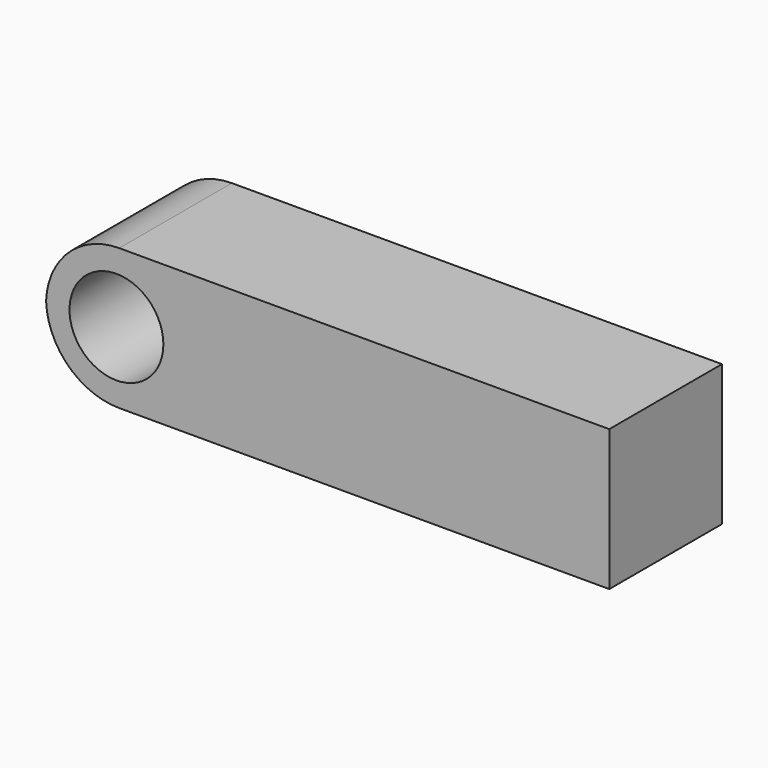
from build123d import *

# Parameters (mm, degrees)
F0_W        = 76.2
F0_H        = 19.05
F1_DEPTH    = 19.05
F3_D        = 12.7
F4_T1_DEPTH = 68.58


# Not quite as in the source:
# - a fillet or chamfer that OpenCascade refuses, or shapes differently, is made with other operations: its cross-section is extruded or revolved along the edge and cut away or added


with BuildPart() as f1:
    # F0 (on Top) → F1 (new body)
    with BuildSketch(Plane.XY):
        with Locations((9.6218887268, -4.4917178258)):
            Rectangle(F0_W, F0_H)
    extrude(amount=F1_DEPTH)

    # F3 (through all)
    with Locations(Plane(origin=(0, 5.0332821742, 0), x_dir=(-1, 0, 0), z_dir=(0, 1, 0))):
        with Locations((18.9531112732, 9.525)):
            Hole(F3_D / 2)

    # F4: fillet of radius 9.906 on 2 edges, made by hand

    # F4_s2 → F4_t1 (cut)
    with BuildSketch(Plane.XZ.offset(-29.7982821742)):
        with BuildLine():
            ThreePointArc((-18.5721112732, 19.05), (-25.5767110476, 16.1485997744), (-28.4781112732, 9.144))
            Line((-28.4781112732, 9.144), (-28.4781112732, 19.05))
            Line((-28.4781112732, 19.05), (-18.5721112732, 19.05))
        make_face()
        with BuildLine():
            ThreePointArc((-18.5721112732, 0), (-25.5767110476, 2.9014002256), (-28.4781112732, 9.906))
            Line((-28.4781112732, 9.906), (-28.4781112732, 0))
            Line((-28.4781112732, 0), (-18.5721112732, 0))
        make_face()
    extrude(amount=F4_T1_DEPTH, mode=Mode.SUBTRACT)


solid = f1.part
